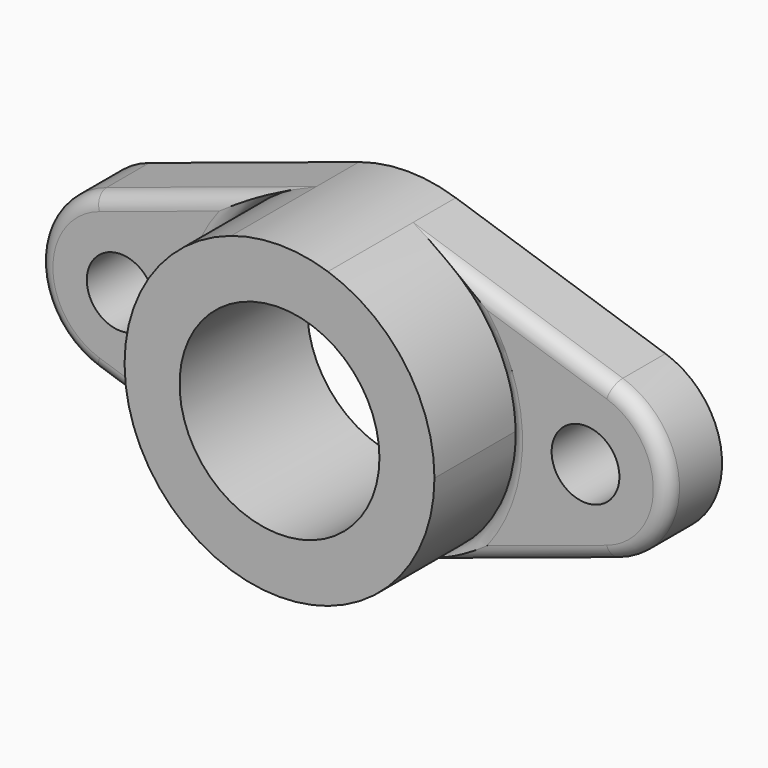
from build123d import *

# Parameters (mm, degrees)
F0_R          = 7
F1_DEPTH      = 14
F0_R_2        = 20.64
F2_DEPTH      = 33
F3_T1_DEPTH   = 68.0960524607
F3_T3_DEPTH   = 68.0960524607
F3_T6_ANGLE   = 224.2346877327
F3_T8_ANGLE   = 143.5800862714
F3_2_T1_DEPTH = 68.0960524607
F3_2_T3_DEPTH = 68.0960524607
F3_2_T6_ANGLE = 224.2346877327
F3_2_T8_ANGLE = 143.5800862714


# Not quite as in the source:
# - a fillet or chamfer that OpenCascade refuses, or shapes differently, is made with other operations: its cross-section is extruded or revolved along the edge and cut away or added


with BuildPart() as f1:
    # F0 (on Front) → F1 (new body)
    with BuildSketch(Plane.XZ):
        with BuildLine():
            ThreePointArc((-10, -30.3973683071), (-32, 0), (-10, 30.3973683071))
            Line((-10, 30.3973683071), (-53.3125, 16.1486019132))
            ThreePointArc((-53.3125, 16.1486019132), (-65, 0), (-53.3125, -16.1486019132))
            Line((-53.3125, -16.1486019132), (-10, -30.3973683071))
        make_face()
        with Locations((-48, 0)):
            Circle(F0_R, mode=Mode.SUBTRACT)
    extrude(amount=F1_DEPTH)

    # F3: fillet of radius 3 on 4 edges, made by hand

    # F3_s2 → F3_t1 (cut)
    with BuildSketch(Plane(origin=(21.373149591, 0, 7.03125), x_dir=(0, 1, 0), z_dir=(-0.9499177596, 0, -0.3125))):
        with BuildLine():
            ThreePointArc((-11, -32), (-13.1213203436, -31.1213203436), (-14, -29))
            Line((-14, -29), (-14, -32))
            Line((-14, -32), (-11, -32))
        make_face()
    extrude(amount=F3_T1_DEPTH, mode=Mode.SUBTRACT)

    # F3_s4 → F3_t3 (cut)
    with BuildSketch(Plane(origin=(-43.3125, 0, 14.248766394), x_dir=(0, 1, 0), z_dir=(0.9499177596, 0, -0.3125))):
        with BuildLine():
            ThreePointArc((-11, -32), (-13.1213203436, -31.1213203436), (-14, -29))
            Line((-14, -29), (-14, -32))
            Line((-14, -32), (-11, -32))
        make_face()
    extrude(amount=F3_T3_DEPTH, mode=Mode.SUBTRACT)

    # F3_s5 → F3_t6 (revolve, cut)
    with BuildSketch(Plane(origin=(0, 0, 0), x_dir=(0, 1, 0), z_dir=(0.9264147025, 0, 0.3765047131))):
        with BuildLine():
            ThreePointArc((-11, -32), (-13.1213203436, -32.8786796564), (-14, -35))
            Line((-14, -35), (-14, -32))
            Line((-14, -32), (-11, -32))
        make_face()
    revolve(axis=Axis((0, -14, 0), (0, 1, 0)), revolution_arc=F3_T6_ANGLE, mode=Mode.SUBTRACT)

    # F3_s7 → F3_t8 (revolve, cut)
    with BuildSketch(Plane(origin=(-43.3125, 0, -14.248766394), x_dir=(0, 1, 0), z_dir=(0.9499177596, 0, 0.3125))):
        with BuildLine():
            ThreePointArc((-11, 32), (-13.1213203436, 31.1213203436), (-14, 29))
            Line((-14, 29), (-14, 32))
            Line((-14, 32), (-11, 32))
        make_face()
    revolve(axis=Axis((-48, -14, 0), (0, -1, 0)), revolution_arc=F3_T8_ANGLE, mode=Mode.SUBTRACT)


with BuildPart() as f1b:
    # F0 (on Front) → F1, piece 2 (new body)
    with BuildSketch(Plane.XZ):
        with BuildLine():
            ThreePointArc((10, 30.3973683071), (25.9229627936, 18.7616630393), (32, 0))
            ThreePointArc((32, 0), (25.9229627936, -18.7616630393), (10, -30.3973683071))
            Line((10, -30.3973683071), (53.3125, -16.1486019132))
            ThreePointArc((53.3125, -16.1486019132), (65, 0), (53.3125, 16.1486019132))
            Line((53.3125, 16.1486019132), (10, 30.3973683071))
        make_face()
        with Locations((48, 0)):
            Circle(F0_R, mode=Mode.SUBTRACT)
    extrude(amount=F1_DEPTH)

    # F3#2: fillet of radius 3 on 4 edges, made by hand

    # F3_2_s2 → F3_2_t1 (cut)
    with BuildSketch(Plane(origin=(43.3125, 0, -14.248766394), x_dir=(0, 1, 0), z_dir=(-0.9499177596, 0, 0.3125))):
        with BuildLine():
            ThreePointArc((-14, -29), (-13.1213203436, -31.1213203436), (-11, -32))
            Line((-11, -32), (-14, -32))
            Line((-14, -32), (-14, -29))
        make_face()
    extrude(amount=F3_2_T1_DEPTH, mode=Mode.SUBTRACT)

    # F3_2_s4 → F3_2_t3 (cut)
    with BuildSketch(Plane(origin=(-21.373149591, 0, -7.03125), x_dir=(0, 1, 0), z_dir=(0.9499177596, 0, 0.3125))):
        with BuildLine():
            ThreePointArc((-14, -29), (-13.1213203436, -31.1213203436), (-11, -32))
            Line((-11, -32), (-14, -32))
            Line((-14, -32), (-14, -29))
        make_face()
    extrude(amount=F3_2_T3_DEPTH, mode=Mode.SUBTRACT)

    # F3_2_s5 → F3_2_t6 (revolve, cut)
    with BuildSketch(Plane(origin=(0, 0, 0), x_dir=(0, 1, 0), z_dir=(-0.9264147025, 0, 0.3765047131))):
        with BuildLine():
            ThreePointArc((-14, 35), (-13.1213203436, 32.8786796564), (-11, 32))
            Line((-11, 32), (-14, 32))
            Line((-14, 32), (-14, 35))
        make_face()
    revolve(axis=Axis((0, -14, 0), (0, -1, 0)), revolution_arc=F3_2_T6_ANGLE, mode=Mode.SUBTRACT)

    # F3_2_s7 → F3_2_t8 (revolve, cut)
    with BuildSketch(Plane(origin=(43.3125, 0, 14.248766394), x_dir=(0, 1, 0), z_dir=(-0.9499177596, 0, -0.3125))):
        with BuildLine():
            ThreePointArc((-11, 32), (-13.1213203436, 31.1213203436), (-14, 29))
            Line((-14, 29), (-14, 32))
            Line((-14, 32), (-11, 32))
        make_face()
    revolve(axis=Axis((48, -14, 0), (0, -1, 0)), revolution_arc=F3_2_T8_ANGLE, mode=Mode.SUBTRACT)


with BuildPart() as f2:
    # F0 (on Front) → F2 (new body)
    with BuildSketch(Plane.XZ):
        with BuildLine():
            ThreePointArc((10, -30.3973683071), (25.9229627936, -18.7616630393), (32, 0))
            ThreePointArc((32, 0), (25.9229627936, 18.7616630393), (10, 30.3973683071))
            ThreePointArc((10, 30.3973683071), (0, 32), (-10, 30.3973683071))
            ThreePointArc((-10, 30.3973683071), (-32, 0), (-10, -30.3973683071))
            ThreePointArc((-10, -30.3973683071), (0, -32), (10, -30.3973683071))
        make_face()
        Circle(F0_R_2, mode=Mode.SUBTRACT)
    extrude(amount=F2_DEPTH)


solid = Compound([f1.part, f1b.part, f2.part])
